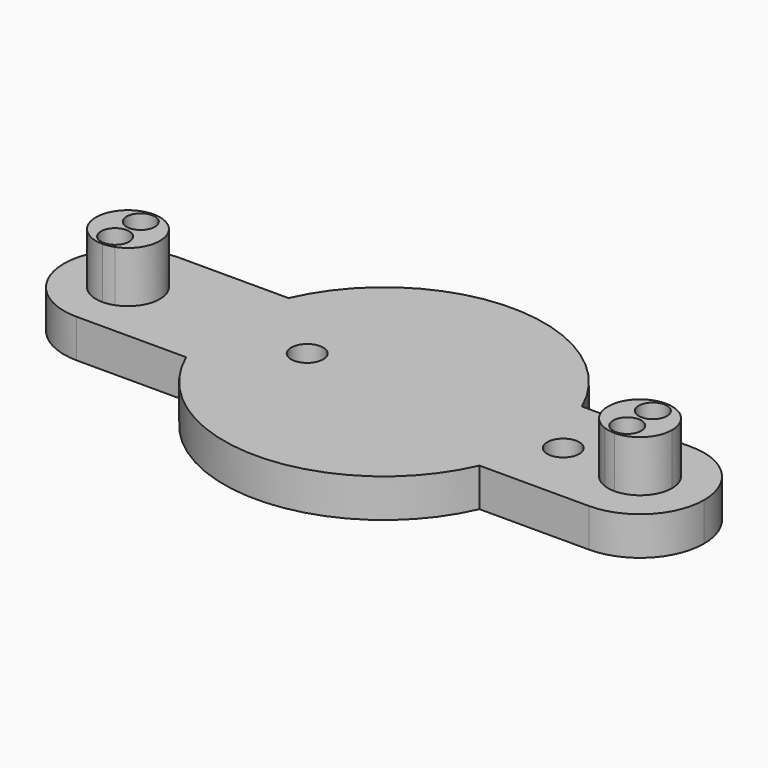
from build123d import *

# Parameters (mm, degrees)
F0_R     = 1.25
F1_DEPTH = 3
F2_DEPTH = 7
F3_DEPTH = 1.5


# Not quite as in the source:
# - a feature names something its author has since deleted; it is built from what else it names


with BuildPart() as f1:
    # F0 (on Top) → F1 (new body)
    with BuildSketch(Plane.XY):
        with BuildLine():
            ThreePointArc((-15, 0), (-15.1488836144, 1.2110614409), (-15.5866679255, 2.35))
            Line((-15.5866679255, 2.35), (-19.1470638945, 2.35))
            ThreePointArc((-19.1470638945, 2.35), (-17.9527652475, 1.4348623168), (-17.5, 0))
            ThreePointArc((-17.5, 0), (-17.9527652475, -1.4348623168), (-19.1470638945, -2.35))
            Line((-19.1470638945, -2.35), (-15.5866679255, -2.35))
            ThreePointArc((-15.5866679255, -2.35), (-15.1488836144, -1.2110614409), (-15, 0))
        make_face()
        with BuildLine():
            Line((-20, -2.5), (-20, -5))
            ThreePointArc((-20, -5), (-17.4260924648, -4.2866070499), (-15.5866679255, -2.35))
            Line((-15.5866679255, -2.35), (-19.1470638945, -2.35))
            ThreePointArc((-19.1470638945, -2.35), (-19.5669872981, -2.4622144504), (-20, -2.5))
        make_face()
        with BuildLine():
            ThreePointArc((-15.5866679255, 2.35), (-17.4260924648, 4.2866070499), (-20, 5))
            Line((-20, 5), (-20, 2.5))
            ThreePointArc((-20, 2.5), (-19.5669872981, 2.4622144504), (-19.1470638945, 2.35))
            Line((-19.1470638945, 2.35), (-15.5866679255, 2.35))
        make_face()
        with BuildLine():
            Line((-20, 2.35), (-20, 2.5))
            ThreePointArc((-20, 2.5), (-22.5, 0), (-20, -2.5))
            Line((-20, -2.5), (-20, -2.35))
            ThreePointArc((-20, -2.35), (-21.1, -1.25), (-20, -0.15))
            Line((-20, -0.15), (-20, 0.15))
            ThreePointArc((-20, 0.15), (-21.1, 1.25), (-20, 2.35))
        make_face()
        with BuildLine():
            ThreePointArc((-12.2771128528, 2.35), (-11.9405191974, 3.6978373809), (-11.4564392374, 5))
            Line((-11.4564392374, 5), (-20, 5))
            ThreePointArc((-20, 5), (-17.4260924648, 4.2866070499), (-15.5866679255, 2.35))
            Line((-15.5866679255, 2.35), (-12.2771128528, 2.35))
        make_face()
        with BuildLine():
            ThreePointArc((-11.4564392374, -5), (-11.9405191974, -3.6978373809), (-12.2771128528, -2.35))
            Line((-12.2771128528, -2.35), (-15.5866679255, -2.35))
            ThreePointArc((-15.5866679255, -2.35), (-17.4260924648, -4.2866070499), (-20, -5))
            Line((-20, -5), (-11.4564392374, -5))
        make_face()
        with BuildLine():
            ThreePointArc((-12.2771128528, -2.35), (-12.5, 0), (-12.2771128528, 2.35))
            Line((-12.2771128528, 2.35), (-15.5866679255, 2.35))
            ThreePointArc((-15.5866679255, 2.35), (-15.1488836144, 1.2110614409), (-15, 0))
            ThreePointArc((-15, 0), (-15.1488836144, -1.2110614409), (-15.5866679255, -2.35))
            Line((-15.5866679255, -2.35), (-12.2771128528, -2.35))
        make_face()
        with BuildLine():
            Line((-11.4564392374, 2.35), (-11.4564392374, 5))
            ThreePointArc((-11.4564392374, 5), (-11.9405191974, 3.6978373809), (-12.2771128528, 2.35))
            Line((-12.2771128528, 2.35), (-11.4564392374, 2.35))
        make_face()
        with BuildLine():
            Line((-11.4564392374, 2.35), (-12.2771128528, 2.35))
            ThreePointArc((-12.2771128528, 2.35), (-12.5, 0), (-12.2771128528, -2.35))
            Line((-12.2771128528, -2.35), (-11.4564392374, -2.35))
            Line((-11.4564392374, -2.35), (-11.4564392374, -1))
            ThreePointArc((-11.4564392374, -1), (-11.5, 0), (-11.4564392374, 1))
            Line((-11.4564392374, 1), (-11.4564392374, 2.35))
        make_face()
        with BuildLine():
            Line((-11.4564392374, -2.35), (-12.2771128528, -2.35))
            ThreePointArc((-12.2771128528, -2.35), (-11.9405191974, -3.6978373809), (-11.4564392374, -5))
            Line((-11.4564392374, -5), (-11.4564392374, -2.35))
        make_face()
        with BuildLine():
            Line((-11.2573309448, 2.35), (-11.4564392374, 2.35))
            Line((-11.4564392374, 2.35), (-11.4564392374, 1))
            ThreePointArc((-11.4564392374, 1), (-11.3769268246, 1.6779559077), (-11.2573309448, 2.35))
        make_face()
        with BuildLine():
            Line((-11.4564392374, -1), (-11.4564392374, -2.35))
            Line((-11.4564392374, -2.35), (-11.2573309448, -2.35))
            ThreePointArc((-11.2573309448, -2.35), (-11.3769268246, -1.6779559077), (-11.4564392374, -1))
        make_face()
        with BuildLine():
            Line((-11.4564392374, -2.35), (-11.4564392374, -5))
            ThreePointArc((-11.4564392374, -5), (0, -12.5), (11.4564392374, -5))
            Line((11.4564392374, -5), (11.4564392374, -2.35))
            Line((11.4564392374, -2.35), (11.2573309448, -2.35))
            ThreePointArc((11.2573309448, -2.35), (0, -11.5), (-11.2573309448, -2.35))
            Line((-11.2573309448, -2.35), (-11.4564392374, -2.35))
        make_face()
        with BuildLine():
            Line((11.4564392374, 2.35), (11.4564392374, 5))
            ThreePointArc((11.4564392374, 5), (0, 12.5), (-11.4564392374, 5))
            Line((-11.4564392374, 5), (-11.4564392374, 2.35))
            Line((-11.4564392374, 2.35), (-11.2573309448, 2.35))
            ThreePointArc((-11.2573309448, 2.35), (0, 11.5), (11.2573309448, 2.35))
            Line((11.2573309448, 2.35), (11.4564392374, 2.35))
        make_face()
        with BuildLine():
            Line((-11.2573309448, 2.35), (11.2573309448, 2.35))
            ThreePointArc((11.2573309448, 2.35), (0, 11.5), (-11.2573309448, 2.35))
        make_face()
        with BuildLine():
            ThreePointArc((-11.2573309448, -2.35), (0, -11.5), (11.2573309448, -2.35))
            Line((11.2573309448, -2.35), (-11.2573309448, -2.35))
        make_face()
        with BuildLine():
            Line((11.4564392374, -1), (11.4564392374, 1))
            ThreePointArc((11.4564392374, 1), (11.3769268246, 1.6779559077), (11.2573309448, 2.35))
            Line((11.2573309448, 2.35), (-11.2573309448, 2.35))
            ThreePointArc((-11.2573309448, 2.35), (-11.3769268246, 1.6779559077), (-11.4564392374, 1))
            Line((-11.4564392374, 1), (-11.4564392374, -1))
            ThreePointArc((-11.4564392374, -1), (-11.3769268246, -1.6779559077), (-11.2573309448, -2.35))
            Line((-11.2573309448, -2.35), (11.2573309448, -2.35))
            ThreePointArc((11.2573309448, -2.35), (11.3769268246, -1.6779559077), (11.4564392374, -1))
        make_face()
        with Locations((-6, 0)):
            Circle(F0_R, mode=Mode.SUBTRACT)
        with BuildLine():
            Line((11.4564392374, 1), (11.4564392374, 2.35))
            Line((11.4564392374, 2.35), (11.2573309448, 2.35))
            ThreePointArc((11.2573309448, 2.35), (11.3769268246, 1.6779559077), (11.4564392374, 1))
        make_face()
        with BuildLine():
            Line((11.4564392374, -2.35), (11.4564392374, -1))
            ThreePointArc((11.4564392374, -1), (11.3769268246, -1.6779559077), (11.2573309448, -2.35))
            Line((11.2573309448, -2.35), (11.4564392374, -2.35))
        make_face()
        with BuildLine():
            ThreePointArc((11.4564392374, -5), (11.9405191974, -3.6978373809), (12.2771128528, -2.35))
            Line((12.2771128528, -2.35), (11.4564392374, -2.35))
            Line((11.4564392374, -2.35), (11.4564392374, -5))
        make_face()
        with BuildLine():
            ThreePointArc((12.2771128528, 2.35), (11.9405191974, 3.6978373809), (11.4564392374, 5))
            Line((11.4564392374, 5), (11.4564392374, 2.35))
            Line((11.4564392374, 2.35), (12.2771128528, 2.35))
        make_face()
        with BuildLine():
            ThreePointArc((12.5, 0), (12.4441534598, 1.1802731337), (12.2771128528, 2.35))
            Line((12.2771128528, 2.35), (11.4564392374, 2.35))
            Line((11.4564392374, 2.35), (11.4564392374, 1))
            ThreePointArc((11.4564392374, 1), (11.4891046481, 0.5004741602), (11.5, 0))
            ThreePointArc((11.5, 0), (11.4891046481, -0.5004741602), (11.4564392374, -1))
            Line((11.4564392374, -1), (11.4564392374, -2.35))
            Line((11.4564392374, -2.35), (12.2771128528, -2.35))
            ThreePointArc((12.2771128528, -2.35), (12.4441534598, -1.1802731337), (12.5, 0))
        make_face()
        with BuildLine():
            Line((20, 5), (11.4564392374, 5))
            ThreePointArc((11.4564392374, 5), (11.9405191974, 3.6978373809), (12.2771128528, 2.35))
            Line((12.2771128528, 2.35), (15.5866679255, 2.35))
            ThreePointArc((15.5866679255, 2.35), (17.4260924648, 4.2866070499), (20, 5))
        make_face()
        with BuildLine():
            Line((15.5866679255, -2.35), (12.2771128528, -2.35))
            ThreePointArc((12.2771128528, -2.35), (11.9405191974, -3.6978373809), (11.4564392374, -5))
            Line((11.4564392374, -5), (20, -5))
            ThreePointArc((20, -5), (17.4260924648, -4.2866070499), (15.5866679255, -2.35))
        make_face()
        with BuildLine():
            Line((15.5866679255, 2.35), (12.2771128528, 2.35))
            ThreePointArc((12.2771128528, 2.35), (12.4441534598, 1.1802731337), (12.5, 0))
            ThreePointArc((12.5, 0), (12.4441534598, -1.1802731337), (12.2771128528, -2.35))
            Line((12.2771128528, -2.35), (15.5866679255, -2.35))
            ThreePointArc((15.5866679255, -2.35), (15.2431824825, -1.5403529158), (15.046875, -0.6830466561))
            ThreePointArc((15.046875, -0.6830466561), (12.75, 0), (15.046875, 0.6830466561))
            ThreePointArc((15.046875, 0.6830466561), (15.2431824825, 1.5403529158), (15.5866679255, 2.35))
        make_face()
        with BuildLine():
            Line((19.1470638945, 2.35), (15.5866679255, 2.35))
            ThreePointArc((15.5866679255, 2.35), (15.2431824825, 1.5403529158), (15.046875, 0.6830466561))
            ThreePointArc((15.046875, 0.6830466561), (15.1981430945, 0.3563048203), (15.25, 0))
            ThreePointArc((15.25, 0), (15.1981430945, -0.3563048203), (15.046875, -0.6830466561))
            ThreePointArc((15.046875, -0.6830466561), (15.2431824825, -1.5403529158), (15.5866679255, -2.35))
            Line((15.5866679255, -2.35), (19.1470638945, -2.35))
            ThreePointArc((19.1470638945, -2.35), (17.5, 0), (19.1470638945, 2.35))
        make_face()
        with BuildLine():
            Line((20, 2.5), (20, 5))
            ThreePointArc((20, 5), (17.4260924648, 4.2866070499), (15.5866679255, 2.35))
            Line((15.5866679255, 2.35), (19.1470638945, 2.35))
            ThreePointArc((19.1470638945, 2.35), (19.5669872981, 2.4622144504), (20, 2.5))
        make_face()
        with BuildLine():
            ThreePointArc((22.5, 0), (21.767766953, 1.767766953), (20, 2.5))
            Line((20, 2.5), (20, 2.35))
            ThreePointArc((20, 2.35), (20.7778174593, 2.0278174593), (21.1, 1.25))
            ThreePointArc((21.1, 1.25), (20.7778174593, 0.4721825407), (20, 0.15))
            Line((20, 0.15), (20, -0.15))
            ThreePointArc((20, -0.15), (20.7778174593, -0.4721825407), (21.1, -1.25))
            ThreePointArc((21.1, -1.25), (20.7778174593, -2.0278174593), (20, -2.35))
            Line((20, -2.35), (20, -2.5))
            ThreePointArc((20, -2.5), (21.767766953, -1.767766953), (22.5, 0))
        make_face()
        with BuildLine():
            ThreePointArc((15.5866679255, -2.35), (17.4260924648, -4.2866070499), (20, -5))
            Line((20, -5), (20, -2.5))
            ThreePointArc((20, -2.5), (19.5669872981, -2.4622144504), (19.1470638945, -2.35))
            Line((19.1470638945, -2.35), (15.5866679255, -2.35))
        make_face()
        with BuildLine():
            Line((-11.4564392374, -1), (-11.4564392374, 1))
            ThreePointArc((-11.4564392374, 1), (-11.5, 0), (-11.4564392374, -1))
        make_face()
        with BuildLine():
            ThreePointArc((11.5, 0), (11.4891046481, 0.5004741602), (11.4564392374, 1))
            Line((11.4564392374, 1), (11.4564392374, -1))
            ThreePointArc((11.4564392374, -1), (11.4891046481, -0.5004741602), (11.5, 0))
        make_face()
        with BuildLine():
            ThreePointArc((25, 0), (23.5355339059, 3.5355339059), (20, 5))
            Line((20, 5), (20, 2.5))
            ThreePointArc((20, 2.5), (21.767766953, 1.767766953), (22.5, 0))
            ThreePointArc((22.5, 0), (21.767766953, -1.767766953), (20, -2.5))
            Line((20, -2.5), (20, -5))
            ThreePointArc((20, -5), (23.5355339059, -3.5355339059), (25, 0))
        make_face()
        with BuildLine():
            Line((-20, 2.5), (-20, 5))
            ThreePointArc((-20, 5), (-25, 0), (-20, -5))
            Line((-20, -5), (-20, -2.5))
            ThreePointArc((-20, -2.5), (-22.5, 0), (-20, 2.5))
        make_face()
        with BuildLine():
            ThreePointArc((-17.5, 0), (-17.9527652475, 1.4348623168), (-19.1470638945, 2.35))
            Line((-19.1470638945, 2.35), (-20, 2.35))
            ThreePointArc((-20, 2.35), (-19.2221825407, 2.0278174593), (-18.9, 1.25))
            ThreePointArc((-18.9, 1.25), (-19.2221825407, 0.4721825407), (-20, 0.15))
            Line((-20, 0.15), (-20, -0.15))
            ThreePointArc((-20, -0.15), (-19.2221825407, -0.4721825407), (-18.9, -1.25))
            ThreePointArc((-18.9, -1.25), (-19.2221825407, -2.0278174593), (-20, -2.35))
            Line((-20, -2.35), (-19.1470638945, -2.35))
            ThreePointArc((-19.1470638945, -2.35), (-17.9527652475, -1.4348623168), (-17.5, 0))
        make_face()
        with BuildLine():
            Line((-20, -2.35), (-20, -2.5))
            ThreePointArc((-20, -2.5), (-19.5669872981, -2.4622144504), (-19.1470638945, -2.35))
            Line((-19.1470638945, -2.35), (-20, -2.35))
        make_face()
        with BuildLine():
            ThreePointArc((-19.1470638945, 2.35), (-19.5669872981, 2.4622144504), (-20, 2.5))
            Line((-20, 2.5), (-20, 2.35))
            Line((-20, 2.35), (-19.1470638945, 2.35))
        make_face()
        with BuildLine():
            Line((20, 2.35), (19.1470638945, 2.35))
            ThreePointArc((19.1470638945, 2.35), (17.5, 0), (19.1470638945, -2.35))
            Line((19.1470638945, -2.35), (20, -2.35))
            ThreePointArc((20, -2.35), (18.9, -1.25), (20, -0.15))
            Line((20, -0.15), (20, 0.15))
            ThreePointArc((20, 0.15), (18.9, 1.25), (20, 2.35))
        make_face()
        with BuildLine():
            Line((20, 2.35), (20, 2.5))
            ThreePointArc((20, 2.5), (19.5669872981, 2.4622144504), (19.1470638945, 2.35))
            Line((19.1470638945, 2.35), (20, 2.35))
        make_face()
        with BuildLine():
            Line((20, -2.35), (19.1470638945, -2.35))
            ThreePointArc((19.1470638945, -2.35), (19.5669872981, -2.4622144504), (20, -2.5))
            Line((20, -2.5), (20, -2.35))
        make_face()
    extrude(amount=F1_DEPTH)

    # F0 (on Top) → F2 (join)
    with BuildSketch(Plane.XY):
        with BuildLine():
            ThreePointArc((-17.5, 0), (-17.9527652475, 1.4348623168), (-19.1470638945, 2.35))
            Line((-19.1470638945, 2.35), (-20, 2.35))
            ThreePointArc((-20, 2.35), (-19.2221825407, 2.0278174593), (-18.9, 1.25))
            ThreePointArc((-18.9, 1.25), (-19.2221825407, 0.4721825407), (-20, 0.15))
            Line((-20, 0.15), (-20, -0.15))
            ThreePointArc((-20, -0.15), (-19.2221825407, -0.4721825407), (-18.9, -1.25))
            ThreePointArc((-18.9, -1.25), (-19.2221825407, -2.0278174593), (-20, -2.35))
            Line((-20, -2.35), (-19.1470638945, -2.35))
            ThreePointArc((-19.1470638945, -2.35), (-17.9527652475, -1.4348623168), (-17.5, 0))
        make_face()
        with BuildLine():
            Line((-20, -2.35), (-20, -2.5))
            ThreePointArc((-20, -2.5), (-19.5669872981, -2.4622144504), (-19.1470638945, -2.35))
            Line((-19.1470638945, -2.35), (-20, -2.35))
        make_face()
        with BuildLine():
            Line((-20, 2.35), (-20, 2.5))
            ThreePointArc((-20, 2.5), (-22.5, 0), (-20, -2.5))
            Line((-20, -2.5), (-20, -2.35))
            ThreePointArc((-20, -2.35), (-21.1, -1.25), (-20, -0.15))
            Line((-20, -0.15), (-20, 0.15))
            ThreePointArc((-20, 0.15), (-21.1, 1.25), (-20, 2.35))
        make_face()
        with BuildLine():
            ThreePointArc((-19.1470638945, 2.35), (-19.5669872981, 2.4622144504), (-20, 2.5))
            Line((-20, 2.5), (-20, 2.35))
            Line((-20, 2.35), (-19.1470638945, 2.35))
        make_face()
        with BuildLine():
            Line((20, -2.35), (19.1470638945, -2.35))
            ThreePointArc((19.1470638945, -2.35), (19.5669872981, -2.4622144504), (20, -2.5))
            Line((20, -2.5), (20, -2.35))
        make_face()
        with BuildLine():
            Line((20, 2.35), (19.1470638945, 2.35))
            ThreePointArc((19.1470638945, 2.35), (17.5, 0), (19.1470638945, -2.35))
            Line((19.1470638945, -2.35), (20, -2.35))
            ThreePointArc((20, -2.35), (18.9, -1.25), (20, -0.15))
            Line((20, -0.15), (20, 0.15))
            ThreePointArc((20, 0.15), (18.9, 1.25), (20, 2.35))
        make_face()
        with BuildLine():
            ThreePointArc((22.5, 0), (21.767766953, 1.767766953), (20, 2.5))
            Line((20, 2.5), (20, 2.35))
            ThreePointArc((20, 2.35), (20.7778174593, 2.0278174593), (21.1, 1.25))
            ThreePointArc((21.1, 1.25), (20.7778174593, 0.4721825407), (20, 0.15))
            Line((20, 0.15), (20, -0.15))
            ThreePointArc((20, -0.15), (20.7778174593, -0.4721825407), (21.1, -1.25))
            ThreePointArc((21.1, -1.25), (20.7778174593, -2.0278174593), (20, -2.35))
            Line((20, -2.35), (20, -2.5))
            ThreePointArc((20, -2.5), (21.767766953, -1.767766953), (22.5, 0))
        make_face()
        with BuildLine():
            Line((20, 2.35), (20, 2.5))
            ThreePointArc((20, 2.5), (19.5669872981, 2.4622144504), (19.1470638945, 2.35))
            Line((19.1470638945, 2.35), (20, 2.35))
        make_face()
    extrude(amount=F2_DEPTH)


with BuildPart() as f3:
    # F0 (on Top) → F3 (new body)
    with BuildSketch(Plane.XY):
        with BuildLine():
            ThreePointArc((-15, 0), (-15.1488836144, 1.2110614409), (-15.5866679255, 2.35))
            Line((-15.5866679255, 2.35), (-19.1470638945, 2.35))
            ThreePointArc((-19.1470638945, 2.35), (-17.9527652475, 1.4348623168), (-17.5, 0))
            ThreePointArc((-17.5, 0), (-17.9527652475, -1.4348623168), (-19.1470638945, -2.35))
            Line((-19.1470638945, -2.35), (-15.5866679255, -2.35))
            ThreePointArc((-15.5866679255, -2.35), (-15.1488836144, -1.2110614409), (-15, 0))
        make_face()
        with BuildLine():
            ThreePointArc((-12.2771128528, -2.35), (-12.5, 0), (-12.2771128528, 2.35))
            Line((-12.2771128528, 2.35), (-15.5866679255, 2.35))
            ThreePointArc((-15.5866679255, 2.35), (-15.1488836144, 1.2110614409), (-15, 0))
            ThreePointArc((-15, 0), (-15.1488836144, -1.2110614409), (-15.5866679255, -2.35))
            Line((-15.5866679255, -2.35), (-12.2771128528, -2.35))
        make_face()
        with BuildLine():
            Line((-11.4564392374, 2.35), (-12.2771128528, 2.35))
            ThreePointArc((-12.2771128528, 2.35), (-12.5, 0), (-12.2771128528, -2.35))
            Line((-12.2771128528, -2.35), (-11.4564392374, -2.35))
            Line((-11.4564392374, -2.35), (-11.4564392374, -1))
            ThreePointArc((-11.4564392374, -1), (-11.5, 0), (-11.4564392374, 1))
            Line((-11.4564392374, 1), (-11.4564392374, 2.35))
        make_face()
        with BuildLine():
            Line((-11.2573309448, 2.35), (-11.4564392374, 2.35))
            Line((-11.4564392374, 2.35), (-11.4564392374, 1))
            ThreePointArc((-11.4564392374, 1), (-11.3769268246, 1.6779559077), (-11.2573309448, 2.35))
        make_face()
        with BuildLine():
            Line((-11.4564392374, -1), (-11.4564392374, -2.35))
            Line((-11.4564392374, -2.35), (-11.2573309448, -2.35))
            ThreePointArc((-11.2573309448, -2.35), (-11.3769268246, -1.6779559077), (-11.4564392374, -1))
        make_face()
        with BuildLine():
            Line((11.4564392374, -1), (11.4564392374, 1))
            ThreePointArc((11.4564392374, 1), (11.3769268246, 1.6779559077), (11.2573309448, 2.35))
            Line((11.2573309448, 2.35), (-11.2573309448, 2.35))
            ThreePointArc((-11.2573309448, 2.35), (-11.3769268246, 1.6779559077), (-11.4564392374, 1))
            Line((-11.4564392374, 1), (-11.4564392374, -1))
            ThreePointArc((-11.4564392374, -1), (-11.3769268246, -1.6779559077), (-11.2573309448, -2.35))
            Line((-11.2573309448, -2.35), (11.2573309448, -2.35))
            ThreePointArc((11.2573309448, -2.35), (11.3769268246, -1.6779559077), (11.4564392374, -1))
        make_face()
        with Locations((-6, 0)):
            Circle(F0_R, mode=Mode.SUBTRACT)
        with BuildLine():
            Line((11.4564392374, 1), (11.4564392374, 2.35))
            Line((11.4564392374, 2.35), (11.2573309448, 2.35))
            ThreePointArc((11.2573309448, 2.35), (11.3769268246, 1.6779559077), (11.4564392374, 1))
        make_face()
        with BuildLine():
            Line((11.4564392374, -2.35), (11.4564392374, -1))
            ThreePointArc((11.4564392374, -1), (11.3769268246, -1.6779559077), (11.2573309448, -2.35))
            Line((11.2573309448, -2.35), (11.4564392374, -2.35))
        make_face()
        with BuildLine():
            ThreePointArc((12.5, 0), (12.4441534598, 1.1802731337), (12.2771128528, 2.35))
            Line((12.2771128528, 2.35), (11.4564392374, 2.35))
            Line((11.4564392374, 2.35), (11.4564392374, 1))
            ThreePointArc((11.4564392374, 1), (11.4891046481, 0.5004741602), (11.5, 0))
            ThreePointArc((11.5, 0), (11.4891046481, -0.5004741602), (11.4564392374, -1))
            Line((11.4564392374, -1), (11.4564392374, -2.35))
            Line((11.4564392374, -2.35), (12.2771128528, -2.35))
            ThreePointArc((12.2771128528, -2.35), (12.4441534598, -1.1802731337), (12.5, 0))
        make_face()
        with BuildLine():
            Line((15.5866679255, 2.35), (12.2771128528, 2.35))
            ThreePointArc((12.2771128528, 2.35), (12.4441534598, 1.1802731337), (12.5, 0))
            ThreePointArc((12.5, 0), (12.4441534598, -1.1802731337), (12.2771128528, -2.35))
            Line((12.2771128528, -2.35), (15.5866679255, -2.35))
            ThreePointArc((15.5866679255, -2.35), (15.2431824825, -1.5403529158), (15.046875, -0.6830466561))
            ThreePointArc((15.046875, -0.6830466561), (12.75, 0), (15.046875, 0.6830466561))
            ThreePointArc((15.046875, 0.6830466561), (15.2431824825, 1.5403529158), (15.5866679255, 2.35))
        make_face()
        with BuildLine():
            Line((19.1470638945, 2.35), (15.5866679255, 2.35))
            ThreePointArc((15.5866679255, 2.35), (15.2431824825, 1.5403529158), (15.046875, 0.6830466561))
            ThreePointArc((15.046875, 0.6830466561), (15.1981430945, 0.3563048203), (15.25, 0))
            ThreePointArc((15.25, 0), (15.1981430945, -0.3563048203), (15.046875, -0.6830466561))
            ThreePointArc((15.046875, -0.6830466561), (15.2431824825, -1.5403529158), (15.5866679255, -2.35))
            Line((15.5866679255, -2.35), (19.1470638945, -2.35))
            ThreePointArc((19.1470638945, -2.35), (17.5, 0), (19.1470638945, 2.35))
        make_face()
        with BuildLine():
            ThreePointArc((11.5, 0), (11.4891046481, 0.5004741602), (11.4564392374, 1))
            Line((11.4564392374, 1), (11.4564392374, -1))
            ThreePointArc((11.4564392374, -1), (11.4891046481, -0.5004741602), (11.5, 0))
        make_face()
        with BuildLine():
            Line((-11.4564392374, -1), (-11.4564392374, 1))
            ThreePointArc((-11.4564392374, 1), (-11.5, 0), (-11.4564392374, -1))
        make_face()
        with BuildLine():
            ThreePointArc((-17.5, 0), (-17.9527652475, 1.4348623168), (-19.1470638945, 2.35))
            Line((-19.1470638945, 2.35), (-20, 2.35))
            ThreePointArc((-20, 2.35), (-19.2221825407, 2.0278174593), (-18.9, 1.25))
            ThreePointArc((-18.9, 1.25), (-19.2221825407, 0.4721825407), (-20, 0.15))
            Line((-20, 0.15), (-20, -0.15))
            ThreePointArc((-20, -0.15), (-19.2221825407, -0.4721825407), (-18.9, -1.25))
            ThreePointArc((-18.9, -1.25), (-19.2221825407, -2.0278174593), (-20, -2.35))
            Line((-20, -2.35), (-19.1470638945, -2.35))
            ThreePointArc((-19.1470638945, -2.35), (-17.9527652475, -1.4348623168), (-17.5, 0))
        make_face()
        with BuildLine():
            Line((20, 2.35), (19.1470638945, 2.35))
            ThreePointArc((19.1470638945, 2.35), (17.5, 0), (19.1470638945, -2.35))
            Line((19.1470638945, -2.35), (20, -2.35))
            ThreePointArc((20, -2.35), (18.9, -1.25), (20, -0.15))
            Line((20, -0.15), (20, 0.15))
            ThreePointArc((20, 0.15), (18.9, 1.25), (20, 2.35))
        make_face()
    extrude(amount=F3_DEPTH)


with BuildPart() as f1_1:
    add(f1.part)

    # F4: cut F3
    add(f3.part, mode=Mode.SUBTRACT)


solid = f1_1.part
